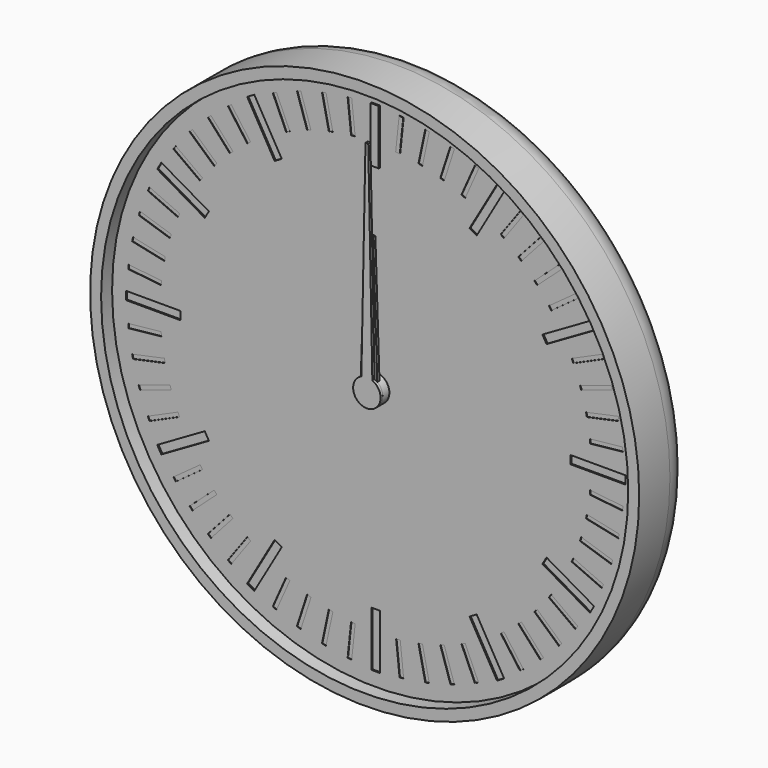
from build123d import *

# Parameters (mm, degrees)
F0_R      = 100
F1_DEPTH  = 24
F2_R      = 10
F3_T      = -4
F4_R      = 5
F4_R_2    = 3
F5_DEPTH  = 2
F6_DEPTH  = 19
F7_DEPTH  = 8
F9_DEPTH  = 4
F11_DEPTH = 4
F12_R     = 5
F12_R_2   = 3
F13_DEPTH = 2
F14_R     = 3
F15_DEPTH = 4
F17_DEPTH = 4
F18_R     = 3
F19_DEPTH = 2
F20_R     = 98
F20_R_2   = 5
F21_DEPTH = 1
F23_R     = 5
F23_R_2   = 3
F24_DEPTH = 2
F25_W     = 3
F25_H     = 20
F25_W_2   = 20
F25_H_2   = 3
F26_DEPTH = 0.5
F27_W     = 1.5
F27_H     = 12
F27_W_2   = 12
F27_H_2   = 1.5
F28_DEPTH = 0.2
F29_DEPTH = 1
F30_DEPTH = 0.4
F31_R     = 5
F31_R_2   = 3
F32_DEPTH = 5
F33_R     = 3
F34_DEPTH = 1
F36_DEPTH = 1


with BuildPart() as f1:
    # F0 (on Front) → F1 (new body)
    with BuildSketch(Plane.XZ):
        Circle(F0_R)
    extrude(amount=F1_DEPTH)

    # F2
    f2_edges = [f1.edges().sort_by_distance(p)[0] for p in [
        (-100, 0, 0),
    ]]
    fillet(f2_edges, radius=F2_R)

    # F3
    f3_openings = [f1.faces().sort_by_distance(p)[0] for p in [
        (0, -24, 0),
    ]]
    offset(amount=F3_T, openings=f3_openings)

    # F4 (on face) → F5 (join)
    with BuildSketch(Plane.XZ.offset(4)):
        Circle(F4_R)
        Circle(F4_R_2, mode=Mode.SUBTRACT)
        with Locations((40, 0)):
            Circle(F4_R)
        with Locations((40, 0)):
            Circle(F4_R_2, mode=Mode.SUBTRACT)
    extrude(amount=F5_DEPTH)


with BuildPart() as f6:
    # F6 (new): a face of the model
    f6_faces = [f1.part.faces().sort_by_distance(p)[0] for p in [
        (0, -4, 0),
    ]]
    extrude(f6_faces, amount=F6_DEPTH)

    # F8 (on face) → F9 (join)
    with BuildSketch(Plane.XZ.offset(6)):
        with BuildLine():
            ThreePointArc((9.2729637667, -1.3794085621), (9.3494561423, -0.6915886375), (9.375, 0))
            ThreePointArc((9.375, 0), (9.3494561423, 0.6915886375), (9.2729637667, 1.3794085621))
            ThreePointArc((9.2729637667, 1.3794085621), (8.9161548403, 2.8970343223), (8.3127812852, 4.3345463782))
            ThreePointArc((8.3127812852, 4.3345463782), (7.5845343223, 5.5104867402), (6.6911892658, 6.566476316))
            ThreePointArc((6.6911892658, 6.566476316), (5.5104867402, 7.5845343223), (4.1773988938, 8.3928519278))
            ThreePointArc((4.1773988938, 8.3928519278), (2.8970343223, 8.9161548403), (1.5536078905, 9.2453733036))
            ThreePointArc((1.5536078905, 9.2453733036), (0, 9.375), (-1.5536078905, 9.2453733036))
            ThreePointArc((-1.5536078905, 9.2453733036), (-2.8970343223, 8.9161548403), (-4.1773988938, 8.3928519278))
            ThreePointArc((-4.1773988938, 8.3928519278), (-5.5104867402, 7.5845343223), (-6.6911892658, 6.566476316))
            ThreePointArc((-6.6911892658, 6.566476316), (-7.5845343223, 5.5104867402), (-8.3127812852, 4.3345463782))
            ThreePointArc((-8.3127812852, 4.3345463782), (-8.9161548403, 2.8970343223), (-9.2729637667, 1.3794085621))
            ThreePointArc((-9.2729637667, 1.3794085621), (-9.375, 0), (-9.2729637667, -1.3794085621))
            ThreePointArc((-9.2729637667, -1.3794085621), (-8.9161548403, -2.8970343223), (-8.3127812852, -4.3345463782))
            ThreePointArc((-8.3127812852, -4.3345463782), (-7.5845343223, -5.5104867402), (-6.6911892658, -6.566476316))
            ThreePointArc((-6.6911892658, -6.566476316), (-5.5104867402, -7.5845343223), (-4.1773988938, -8.3928519278))
            ThreePointArc((-4.1773988938, -8.3928519278), (-2.8970343223, -8.9161548403), (-1.5536078905, -9.2453733036))
            ThreePointArc((-1.5536078905, -9.2453733036), (0, -9.375), (1.5536078905, -9.2453733036))
            ThreePointArc((1.5536078905, -9.2453733036), (2.8970343223, -8.9161548403), (4.1773988938, -8.3928519278))
            ThreePointArc((4.1773988938, -8.3928519278), (5.5104867402, -7.5845343223), (6.6911892658, -6.566476316))
            ThreePointArc((6.6911892658, -6.566476316), (7.5845343223, -5.5104867402), (8.3127812852, -4.3345463782))
            ThreePointArc((8.3127812852, -4.3345463782), (8.9161548403, -2.8970343223), (9.2729637667, -1.3794085621))
        make_face()
        with BuildLine():
            ThreePointArc((8.3127812852, 4.3345463782), (8.9161548403, 2.8970343223), (9.2729637667, 1.3794085621))
            Line((9.2729637667, 1.3794085621), (11.1823199426, 2.3946312492))
            Line((11.1823199426, 2.3946312492), (10.8182678729, 3.515068311))
            Line((10.8182678729, 3.515068311), (10.4542158031, 4.6355053728))
            Line((10.4542158031, 4.6355053728), (8.3127812852, 4.3345463782))
        make_face()
        with BuildLine():
            Line((11.1823199426, -2.3946312492), (9.2729637667, -1.3794085621))
            ThreePointArc((9.2729637667, -1.3794085621), (8.9161548403, -2.8970343223), (8.3127812852, -4.3345463782))
            Line((8.3127812852, -4.3345463782), (10.4542158031, -4.6355053728))
            Line((10.4542158031, -4.6355053728), (10.8182678729, -3.515068311))
            Line((10.8182678729, -3.515068311), (11.1823199426, -2.3946312492))
        make_face()
        with BuildLine():
            ThreePointArc((4.1773988938, 8.3928519278), (5.5104867402, 7.5845343223), (6.6911892658, 6.566476316))
            Line((6.6911892658, 6.566476316), (7.6391579371, 8.5101001246))
            Line((7.6391579371, 8.5101001246), (6.6860572448, 9.202568311))
            Line((6.6860572448, 9.202568311), (5.7329565525, 9.8950364974))
            Line((5.7329565525, 9.8950364974), (4.1773988938, 8.3928519278))
        make_face()
        with BuildLine():
            Line((7.6391579371, -8.5101001246), (6.6911892658, -6.566476316))
            ThreePointArc((6.6911892658, -6.566476316), (5.5104867402, -7.5845343223), (4.1773988938, -8.3928519278))
            Line((4.1773988938, -8.3928519278), (5.7329565525, -9.8950364974))
            Line((5.7329565525, -9.8950364974), (6.6860572448, -9.202568311))
            Line((6.6860572448, -9.202568311), (7.6391579371, -8.5101001246))
        make_face()
        with BuildLine():
            ThreePointArc((-1.5536078905, 9.2453733036), (0, 9.375), (1.5536078905, 9.2453733036))
            Line((1.5536078905, 9.2453733036), (1.1780972451, 11.375))
            Line((1.1780972451, 11.375), (0, 11.375))
            Line((0, 11.375), (-1.1780972451, 11.375))
            Line((-1.1780972451, 11.375), (-1.5536078905, 9.2453733036))
        make_face()
        with BuildLine():
            Line((1.1780972451, -11.375), (1.5536078905, -9.2453733036))
            ThreePointArc((1.5536078905, -9.2453733036), (0, -9.375), (-1.5536078905, -9.2453733036))
            Line((-1.5536078905, -9.2453733036), (-1.1780972451, -11.375))
            Line((-1.1780972451, -11.375), (0, -11.375))
            Line((0, -11.375), (1.1780972451, -11.375))
        make_face()
        with BuildLine():
            ThreePointArc((-6.6911892658, 6.566476316), (-5.5104867402, 7.5845343223), (-4.1773988938, 8.3928519278))
            Line((-4.1773988938, 8.3928519278), (-5.7329565525, 9.8950364974))
            Line((-5.7329565525, 9.8950364974), (-6.6860572448, 9.202568311))
            Line((-6.6860572448, 9.202568311), (-7.6391579371, 8.5101001246))
            Line((-7.6391579371, 8.5101001246), (-6.6911892658, 6.566476316))
        make_face()
        with BuildLine():
            Line((-5.7329565525, -9.8950364974), (-4.1773988938, -8.3928519278))
            ThreePointArc((-4.1773988938, -8.3928519278), (-5.5104867402, -7.5845343223), (-6.6911892658, -6.566476316))
            Line((-6.6911892658, -6.566476316), (-7.6391579371, -8.5101001246))
            Line((-7.6391579371, -8.5101001246), (-6.6860572448, -9.202568311))
            Line((-6.6860572448, -9.202568311), (-5.7329565525, -9.8950364974))
        make_face()
        with BuildLine():
            ThreePointArc((-9.2729637667, 1.3794085621), (-8.9161548403, 2.8970343223), (-8.3127812852, 4.3345463782))
            Line((-8.3127812852, 4.3345463782), (-10.4542158031, 4.6355053728))
            Line((-10.4542158031, 4.6355053728), (-10.8182678729, 3.515068311))
            Line((-10.8182678729, 3.515068311), (-11.1823199426, 2.3946312492))
            Line((-11.1823199426, 2.3946312492), (-9.2729637667, 1.3794085621))
        make_face()
        with BuildLine():
            Line((-10.4542158031, -4.6355053728), (-8.3127812852, -4.3345463782))
            ThreePointArc((-8.3127812852, -4.3345463782), (-8.9161548403, -2.8970343223), (-9.2729637667, -1.3794085621))
            Line((-9.2729637667, -1.3794085621), (-11.1823199426, -2.3946312492))
            Line((-11.1823199426, -2.3946312492), (-10.8182678729, -3.515068311))
            Line((-10.8182678729, -3.515068311), (-10.4542158031, -4.6355053728))
        make_face()
    extrude(amount=F9_DEPTH)

    # F35 (on face) → F36 (join)
    with BuildSketch(Plane.XZ.offset(23)):
        with BuildLine():
            ThreePointArc((-2, 4.582575695), (-2.7386127875, -4.1833001327), (5, 0))
            ThreePointArc((5, 0), (4.1833001327, 2.7386127875), (2, 4.582575695))
            ThreePointArc((2, 4.582575695), (0, 5), (-2, 4.582575695))
        make_face()
        with BuildLine():
            ThreePointArc((-2, 4.582575695), (0, 5), (2, 4.582575695))
            Line((2, 4.582575695), (0.5, 80))
            Line((0.5, 80), (0, 80))
            Line((0, 80), (-0.5, 80))
            Line((-0.5, 80), (-2, 4.582575695))
        make_face()
    extrude(amount=-F36_DEPTH)


with BuildPart() as f7:
    # F7 (new): a face of the model
    f7_faces = [f1.part.faces().sort_by_distance(p)[0] for p in [
        (40, -4, 0),
    ]]
    extrude(f7_faces, amount=F7_DEPTH)

    # F10 (on face) → F11 (join)
    with BuildSketch(Plane.XZ.offset(6)):
        with BuildLine():
            ThreePointArc((68.0829066802, -1.5381733945), (68.1144747006, -0.7693746225), (68.125, 0))
            ThreePointArc((68.125, 0), (68.1144747006, 0.7693746225), (68.0829066802, 1.5381733945))
            ThreePointArc((68.0829066802, 1.5381733945), (67.9709283072, 2.9398630294), (67.7890320221, 4.3342039956))
            ThreePointArc((67.7890320221, 4.3342039956), (67.5104012706, 5.8475163042), (67.1494235596, 7.3433252263))
            ThreePointArc((67.1494235596, 7.3433252263), (66.7484645208, 8.6911029668), (66.280643318, 10.0171558733))
            ThreePointArc((66.280643318, 10.0171558733), (65.6934659962, 11.4394680865), (65.0293803521, 12.8275385085))
            ThreePointArc((65.0293803521, 12.8275385085), (64.3569644814, 14.0625), (63.6236643925, 15.2623099717))
            ThreePointArc((63.6236643925, 15.2623099717), (62.7536029668, 16.5314602207), (61.815433119, 17.7511268046))
            ThreePointArc((61.815433119, 17.7511268046), (60.9009482166, 18.8192983038), (59.934217974, 19.8404278876))
            ThreePointArc((59.934217974, 19.8404278876), (58.8192983038, 20.9009482166), (57.6480467764, 21.8989056799))
            ThreePointArc((57.6480467764, 21.8989056799), (56.5314602207, 22.7536029668), (55.3735505752, 23.5514238999))
            ThreePointArc((55.3735505752, 23.5514238999), (54.0625, 24.3569644814), (52.709356105, 25.0895972944))
            ThreePointArc((52.709356105, 25.0895972944), (51.4394680865, 25.6934659962), (50.1409852457, 26.2331096755))
            ThreePointArc((50.1409852457, 26.2331096755), (48.6911029668, 26.7484645208), (47.2152055856, 27.1837531139))
            ThreePointArc((47.2152055856, 27.1837531139), (45.8475163042, 27.5104012706), (44.4652101991, 27.7682826779))
            ThreePointArc((44.4652101991, 27.7682826779), (42.9398630294, 27.9709283072), (41.4057159597, 28.0898484802))
            ThreePointArc((41.4057159597, 28.0898484802), (40, 28.125), (38.5942840403, 28.0898484802))
            ThreePointArc((38.5942840403, 28.0898484802), (37.0601369706, 27.9709283072), (35.5347898009, 27.7682826779))
            ThreePointArc((35.5347898009, 27.7682826779), (34.1524836958, 27.5104012706), (32.7847944144, 27.1837531139))
            ThreePointArc((32.7847944144, 27.1837531139), (31.3088970332, 26.7484645208), (29.8590147543, 26.2331096755))
            ThreePointArc((29.8590147543, 26.2331096755), (28.5605319135, 25.6934659962), (27.290643895, 25.0895972944))
            ThreePointArc((27.290643895, 25.0895972944), (25.9375, 24.3569644814), (24.6264494248, 23.5514238999))
            ThreePointArc((24.6264494248, 23.5514238999), (23.4685397793, 22.7536029668), (22.3519532236, 21.8989056799))
            ThreePointArc((22.3519532236, 21.8989056799), (21.1807016962, 20.9009482166), (20.065782026, 19.8404278876))
            ThreePointArc((20.065782026, 19.8404278876), (19.0990517834, 18.8192983038), (18.184566881, 17.7511268046))
            ThreePointArc((18.184566881, 17.7511268046), (17.2463970332, 16.5314602207), (16.3763356075, 15.2623099717))
            ThreePointArc((16.3763356075, 15.2623099717), (15.6430355186, 14.0625), (14.9706196479, 12.8275385085))
            ThreePointArc((14.9706196479, 12.8275385085), (14.3065340038, 11.4394680865), (13.719356682, 10.0171558733))
            ThreePointArc((13.719356682, 10.0171558733), (13.2515354792, 8.6911029668), (12.8505764404, 7.3433252263))
            ThreePointArc((12.8505764404, 7.3433252263), (12.4895987294, 5.8475163042), (12.2109679779, 4.3342039956))
            ThreePointArc((12.2109679779, 4.3342039956), (12.0290716928, 2.9398630294), (11.9170933198, 1.5381733945))
            ThreePointArc((11.9170933198, 1.5381733945), (11.875, 0), (11.9170933198, -1.5381733945))
            ThreePointArc((11.9170933198, -1.5381733945), (12.0290716928, -2.9398630294), (12.2109679779, -4.3342039956))
            ThreePointArc((12.2109679779, -4.3342039956), (12.4895987294, -5.8475163042), (12.8505764404, -7.3433252263))
            ThreePointArc((12.8505764404, -7.3433252263), (13.2515354792, -8.6911029668), (13.719356682, -10.0171558733))
            ThreePointArc((13.719356682, -10.0171558733), (14.3065340038, -11.4394680865), (14.9706196479, -12.8275385085))
            ThreePointArc((14.9706196479, -12.8275385085), (15.6430355186, -14.0625), (16.3763356075, -15.2623099717))
            ThreePointArc((16.3763356075, -15.2623099717), (17.2463970332, -16.5314602207), (18.184566881, -17.7511268046))
            ThreePointArc((18.184566881, -17.7511268046), (19.0990517834, -18.8192983038), (20.065782026, -19.8404278876))
            ThreePointArc((20.065782026, -19.8404278876), (21.1807016962, -20.9009482166), (22.3519532236, -21.8989056799))
            ThreePointArc((22.3519532236, -21.8989056799), (23.4685397793, -22.7536029668), (24.6264494248, -23.5514238999))
            ThreePointArc((24.6264494248, -23.5514238999), (25.9375, -24.3569644814), (27.290643895, -25.0895972944))
            ThreePointArc((27.290643895, -25.0895972944), (28.5605319135, -25.6934659962), (29.8590147543, -26.2331096755))
            ThreePointArc((29.8590147543, -26.2331096755), (31.3088970332, -26.7484645208), (32.7847944144, -27.1837531139))
            ThreePointArc((32.7847944144, -27.1837531139), (34.1524836958, -27.5104012706), (35.5347898009, -27.7682826779))
            ThreePointArc((35.5347898009, -27.7682826779), (37.0601369706, -27.9709283072), (38.5942840403, -28.0898484802))
            ThreePointArc((38.5942840403, -28.0898484802), (40, -28.125), (41.4057159597, -28.0898484802))
            ThreePointArc((41.4057159597, -28.0898484802), (42.9398630294, -27.9709283072), (44.4652101991, -27.7682826779))
            ThreePointArc((44.4652101991, -27.7682826779), (45.8475163042, -27.5104012706), (47.2152055856, -27.1837531139))
            ThreePointArc((47.2152055856, -27.1837531139), (48.6911029668, -26.7484645208), (50.1409852457, -26.2331096755))
            ThreePointArc((50.1409852457, -26.2331096755), (51.4394680865, -25.6934659962), (52.709356105, -25.0895972944))
            ThreePointArc((52.709356105, -25.0895972944), (54.0625, -24.3569644814), (55.3735505752, -23.5514238999))
            ThreePointArc((55.3735505752, -23.5514238999), (56.5314602207, -22.7536029668), (57.6480467764, -21.8989056799))
            ThreePointArc((57.6480467764, -21.8989056799), (58.8192983038, -20.9009482166), (59.934217974, -19.8404278876))
            ThreePointArc((59.934217974, -19.8404278876), (60.9009482166, -18.8192983038), (61.815433119, -17.7511268046))
            ThreePointArc((61.815433119, -17.7511268046), (62.7536029668, -16.5314602207), (63.6236643925, -15.2623099717))
            ThreePointArc((63.6236643925, -15.2623099717), (64.3569644814, -14.0625), (65.0293803521, -12.8275385085))
            ThreePointArc((65.0293803521, -12.8275385085), (65.6934659962, -11.4394680865), (66.280643318, -10.0171558733))
            ThreePointArc((66.280643318, -10.0171558733), (66.7484645208, -8.6911029668), (67.1494235596, -7.3433252263))
            ThreePointArc((67.1494235596, -7.3433252263), (67.5104012706, -5.8475163042), (67.7890320221, -4.3342039956))
            ThreePointArc((67.7890320221, -4.3342039956), (67.9709283072, -2.9398630294), (68.0829066802, -1.5381733945))
        make_face()
        with BuildLine():
            ThreePointArc((68.0829066802, 1.5381733945), (68.1144747006, 0.7693746225), (68.125, 0))
            ThreePointArc((68.125, 0), (68.1144747006, -0.7693746225), (68.0829066802, -1.5381733945))
            Line((68.0829066802, -1.5381733945), (70.125, -1.1780972451))
            Line((70.125, -1.1780972451), (70.125, 0))
            Line((70.125, 0), (70.125, 1.1780972451))
            Line((70.125, 1.1780972451), (68.0829066802, 1.5381733945))
        make_face()
        with BuildLine():
            ThreePointArc((67.1494235596, 7.3433252263), (67.5104012706, 5.8475163042), (67.7890320221, 4.3342039956))
            Line((67.7890320221, 4.3342039956), (69.7116366623, 5.1109866922))
            Line((69.7116366623, 5.1109866922), (69.4666964721, 6.2633396859))
            Line((69.4666964721, 6.2633396859), (69.2217562819, 7.4156926796))
            Line((69.2217562819, 7.4156926796), (67.1494235596, 7.3433252263))
        make_face()
        with BuildLine():
            Line((69.7116366623, -5.1109866922), (67.7890320221, -4.3342039956))
            ThreePointArc((67.7890320221, -4.3342039956), (67.5104012706, -5.8475163042), (67.1494235596, -7.3433252263))
            Line((67.1494235596, -7.3433252263), (69.2217562819, -7.4156926796))
            Line((69.2217562819, -7.4156926796), (69.4666964721, -6.2633396859))
            Line((69.4666964721, -6.2633396859), (69.7116366623, -5.1109866922))
        make_face()
        with BuildLine():
            ThreePointArc((65.0293803521, 12.8275385085), (65.6934659962, 11.4394680865), (66.280643318, 10.0171558733))
            Line((66.280643318, 10.0171558733), (67.9997322302, 11.1766959857))
            Line((67.9997322302, 11.1766959857), (67.5205569115, 12.2529413727))
            Line((67.5205569115, 12.2529413727), (67.0413815928, 13.3291867596))
            Line((67.0413815928, 13.3291867596), (65.0293803521, 12.8275385085))
        make_face()
        with BuildLine():
            Line((67.9997322302, -11.1766959857), (66.280643318, -10.0171558733))
            ThreePointArc((66.280643318, -10.0171558733), (65.6934659962, -11.4394680865), (65.0293803521, -12.8275385085))
            Line((65.0293803521, -12.8275385085), (67.0413815928, -13.3291867596))
            Line((67.0413815928, -13.3291867596), (67.5205569115, -12.2529413727))
            Line((67.5205569115, -12.2529413727), (67.9997322302, -11.1766959857))
        make_face()
        with BuildLine():
            ThreePointArc((61.815433119, 17.7511268046), (62.7536029668, 16.5314602207), (63.6236643925, 15.2623099717))
            Line((63.6236643925, 15.2623099717), (65.064105142, 16.753930033))
            Line((65.064105142, 16.753930033), (64.3716369555, 17.7070307253))
            Line((64.3716369555, 17.7070307253), (63.6791687691, 18.6601314176))
            Line((63.6791687691, 18.6601314176), (61.815433119, 17.7511268046))
        make_face()
        with BuildLine():
            Line((65.064105142, -16.753930033), (63.6236643925, -15.2623099717))
            ThreePointArc((63.6236643925, -15.2623099717), (62.7536029668, -16.5314602207), (61.815433119, -17.7511268046))
            Line((61.815433119, -17.7511268046), (63.6791687691, -18.6601314176))
            Line((63.6791687691, -18.6601314176), (64.3716369555, -17.7070307253))
            Line((64.3716369555, -17.7070307253), (65.064105142, -16.753930033))
        make_face()
        with BuildLine():
            ThreePointArc((57.6480467764, 21.8989056799), (58.8192983038, 20.9009482166), (59.934217974, 19.8404278876))
            Line((59.934217974, 19.8404278876), (61.0330563882, 21.5989369435))
            Line((61.0330563882, 21.5989369435), (60.1575595166, 22.3872378675))
            Line((60.1575595166, 22.3872378675), (59.282062645, 23.1755387915))
            Line((59.282062645, 23.1755387915), (57.6480467764, 21.8989056799))
        make_face()
        with BuildLine():
            Line((61.0330563882, -21.5989369435), (59.934217974, -19.8404278876))
            ThreePointArc((59.934217974, -19.8404278876), (58.8192983038, -20.9009482166), (57.6480467764, -21.8989056799))
            Line((57.6480467764, -21.8989056799), (59.282062645, -23.1755387915))
            Line((59.282062645, -23.1755387915), (60.1575595166, -22.3872378675))
            Line((60.1575595166, -22.3872378675), (61.0330563882, -21.5989369435))
        make_face()
        with BuildLine():
            ThreePointArc((52.709356105, 25.0895972944), (54.0625, 24.3569644814), (55.3735505752, 23.5514238999))
            Line((55.3735505752, 23.5514238999), (56.0827621424, 25.4999666665))
            Line((56.0827621424, 25.4999666665), (55.0625, 26.089015289))
            Line((55.0625, 26.089015289), (54.0422378576, 26.6780639116))
            Line((54.0422378576, 26.6780639116), (52.709356105, 25.0895972944))
        make_face()
        with BuildLine():
            Line((56.0827621424, -25.4999666665), (55.3735505752, -23.5514238999))
            ThreePointArc((55.3735505752, -23.5514238999), (54.0625, -24.3569644814), (52.709356105, -25.0895972944))
            Line((52.709356105, -25.0895972944), (54.0422378576, -26.6780639116))
            Line((54.0422378576, -26.6780639116), (55.0625, -26.089015289))
            Line((55.0625, -26.089015289), (56.0827621424, -25.4999666665))
        make_face()
        with BuildLine():
            ThreePointArc((47.2152055856, 27.1837531139), (48.6911029668, 26.7484645208), (50.1409852457, 26.2331096755))
            Line((50.1409852457, 26.2331096755), (50.4295740173, 28.2865254836))
            Line((50.4295740173, 28.2865254836), (49.3091369555, 28.6505775534))
            Line((49.3091369555, 28.6505775534), (48.1886998938, 29.0146296232))
            Line((48.1886998938, 29.0146296232), (47.2152055856, 27.1837531139))
        make_face()
        with BuildLine():
            Line((50.4295740173, -28.2865254836), (50.1409852457, -26.2331096755))
            ThreePointArc((50.1409852457, -26.2331096755), (48.6911029668, -26.7484645208), (47.2152055856, -27.1837531139))
            Line((47.2152055856, -27.1837531139), (48.1886998938, -29.0146296232))
            Line((48.1886998938, -29.0146296232), (49.3091369555, -28.6505775534))
            Line((49.3091369555, -28.6505775534), (50.4295740173, -28.2865254836))
        make_face()
        with BuildLine():
            ThreePointArc((41.4057159597, 28.0898484802), (42.9398630294, 27.9709283072), (44.4652101991, 27.7682826779))
            Line((44.4652101991, 27.7682826779), (44.3205634611, 29.8368274034))
            Line((44.3205634611, 29.8368274034), (43.1489199559, 29.959972098))
            Line((43.1489199559, 29.959972098), (41.9772764508, 30.0831167926))
            Line((41.9772764508, 30.0831167926), (41.4057159597, 28.0898484802))
        make_face()
        with BuildLine():
            Line((44.3205634611, -29.8368274034), (44.4652101991, -27.7682826779))
            ThreePointArc((44.4652101991, -27.7682826779), (42.9398630294, -27.9709283072), (41.4057159597, -28.0898484802))
            Line((41.4057159597, -28.0898484802), (41.9772764508, -30.0831167926))
            Line((41.9772764508, -30.0831167926), (43.1489199559, -29.959972098))
            Line((43.1489199559, -29.959972098), (44.3205634611, -29.8368274034))
        make_face()
        with BuildLine():
            ThreePointArc((35.5347898009, 27.7682826779), (37.0601369706, 27.9709283072), (38.5942840403, 28.0898484802))
            Line((38.5942840403, 28.0898484802), (38.0227235492, 30.0831167926))
            Line((38.0227235492, 30.0831167926), (36.8510800441, 29.959972098))
            Line((36.8510800441, 29.959972098), (35.6794365389, 29.8368274034))
            Line((35.6794365389, 29.8368274034), (35.5347898009, 27.7682826779))
        make_face()
        with BuildLine():
            Line((38.0227235492, -30.0831167926), (38.5942840403, -28.0898484802))
            ThreePointArc((38.5942840403, -28.0898484802), (37.0601369706, -27.9709283072), (35.5347898009, -27.7682826779))
            Line((35.5347898009, -27.7682826779), (35.6794365389, -29.8368274034))
            Line((35.6794365389, -29.8368274034), (36.8510800441, -29.959972098))
            Line((36.8510800441, -29.959972098), (38.0227235492, -30.0831167926))
        make_face()
        with BuildLine():
            ThreePointArc((29.8590147543, 26.2331096755), (31.3088970332, 26.7484645208), (32.7847944144, 27.1837531139))
            Line((32.7847944144, 27.1837531139), (31.8113001062, 29.0146296232))
            Line((31.8113001062, 29.0146296232), (30.6908630445, 28.6505775534))
            Line((30.6908630445, 28.6505775534), (29.5704259827, 28.2865254836))
            Line((29.5704259827, 28.2865254836), (29.8590147543, 26.2331096755))
        make_face()
        with BuildLine():
            Line((31.8113001062, -29.0146296232), (32.7847944144, -27.1837531139))
            ThreePointArc((32.7847944144, -27.1837531139), (31.3088970332, -26.7484645208), (29.8590147543, -26.2331096755))
            Line((29.8590147543, -26.2331096755), (29.5704259827, -28.2865254836))
            Line((29.5704259827, -28.2865254836), (30.6908630445, -28.6505775534))
            Line((30.6908630445, -28.6505775534), (31.8113001062, -29.0146296232))
        make_face()
        with BuildLine():
            ThreePointArc((24.6264494248, 23.5514238999), (25.9375, 24.3569644814), (27.290643895, 25.0895972944))
            Line((27.290643895, 25.0895972944), (25.9577621424, 26.6780639116))
            Line((25.9577621424, 26.6780639116), (24.9375, 26.089015289))
            Line((24.9375, 26.089015289), (23.9172378576, 25.4999666665))
            Line((23.9172378576, 25.4999666665), (24.6264494248, 23.5514238999))
        make_face()
        with BuildLine():
            Line((25.9577621424, -26.6780639116), (27.290643895, -25.0895972944))
            ThreePointArc((27.290643895, -25.0895972944), (25.9375, -24.3569644814), (24.6264494248, -23.5514238999))
            Line((24.6264494248, -23.5514238999), (23.9172378576, -25.4999666665))
            Line((23.9172378576, -25.4999666665), (24.9375, -26.089015289))
            Line((24.9375, -26.089015289), (25.9577621424, -26.6780639116))
        make_face()
        with BuildLine():
            ThreePointArc((20.065782026, 19.8404278876), (21.1807016962, 20.9009482166), (22.3519532236, 21.8989056799))
            Line((22.3519532236, 21.8989056799), (20.717937355, 23.1755387915))
            Line((20.717937355, 23.1755387915), (19.8424404834, 22.3872378675))
            Line((19.8424404834, 22.3872378675), (18.9669436118, 21.5989369435))
            Line((18.9669436118, 21.5989369435), (20.065782026, 19.8404278876))
        make_face()
        with BuildLine():
            Line((20.717937355, -23.1755387915), (22.3519532236, -21.8989056799))
            ThreePointArc((22.3519532236, -21.8989056799), (21.1807016962, -20.9009482166), (20.065782026, -19.8404278876))
            Line((20.065782026, -19.8404278876), (18.9669436118, -21.5989369435))
            Line((18.9669436118, -21.5989369435), (19.8424404834, -22.3872378675))
            Line((19.8424404834, -22.3872378675), (20.717937355, -23.1755387915))
        make_face()
        with BuildLine():
            ThreePointArc((16.3763356075, 15.2623099717), (17.2463970332, 16.5314602207), (18.184566881, 17.7511268046))
            Line((18.184566881, 17.7511268046), (16.3208312309, 18.6601314176))
            Line((16.3208312309, 18.6601314176), (15.6283630445, 17.7070307253))
            Line((15.6283630445, 17.7070307253), (14.935894858, 16.753930033))
            Line((14.935894858, 16.753930033), (16.3763356075, 15.2623099717))
        make_face()
        with BuildLine():
            Line((16.3208312309, -18.6601314176), (18.184566881, -17.7511268046))
            ThreePointArc((18.184566881, -17.7511268046), (17.2463970332, -16.5314602207), (16.3763356075, -15.2623099717))
            Line((16.3763356075, -15.2623099717), (14.935894858, -16.753930033))
            Line((14.935894858, -16.753930033), (15.6283630445, -17.7070307253))
            Line((15.6283630445, -17.7070307253), (16.3208312309, -18.6601314176))
        make_face()
        with BuildLine():
            ThreePointArc((13.719356682, 10.0171558733), (14.3065340038, 11.4394680865), (14.9706196479, 12.8275385085))
            Line((14.9706196479, 12.8275385085), (12.9586184072, 13.3291867596))
            Line((12.9586184072, 13.3291867596), (12.4794430885, 12.2529413727))
            Line((12.4794430885, 12.2529413727), (12.0002677698, 11.1766959857))
            Line((12.0002677698, 11.1766959857), (13.719356682, 10.0171558733))
        make_face()
        with BuildLine():
            Line((12.9586184072, -13.3291867596), (14.9706196479, -12.8275385085))
            ThreePointArc((14.9706196479, -12.8275385085), (14.3065340038, -11.4394680865), (13.719356682, -10.0171558733))
            Line((13.719356682, -10.0171558733), (12.0002677698, -11.1766959857))
            Line((12.0002677698, -11.1766959857), (12.4794430885, -12.2529413727))
            Line((12.4794430885, -12.2529413727), (12.9586184072, -13.3291867596))
        make_face()
        with BuildLine():
            ThreePointArc((12.2109679779, 4.3342039956), (12.4895987294, 5.8475163042), (12.8505764404, 7.3433252263))
            Line((12.8505764404, 7.3433252263), (10.7782437181, 7.4156926796))
            Line((10.7782437181, 7.4156926796), (10.5333035279, 6.2633396859))
            Line((10.5333035279, 6.2633396859), (10.2883633377, 5.1109866922))
            Line((10.2883633377, 5.1109866922), (12.2109679779, 4.3342039956))
        make_face()
        with BuildLine():
            Line((10.7782437181, -7.4156926796), (12.8505764404, -7.3433252263))
            ThreePointArc((12.8505764404, -7.3433252263), (12.4895987294, -5.8475163042), (12.2109679779, -4.3342039956))
            Line((12.2109679779, -4.3342039956), (10.2883633377, -5.1109866922))
            Line((10.2883633377, -5.1109866922), (10.5333035279, -6.2633396859))
            Line((10.5333035279, -6.2633396859), (10.7782437181, -7.4156926796))
        make_face()
        with BuildLine():
            ThreePointArc((11.9170933198, -1.5381733945), (11.875, 0), (11.9170933198, 1.5381733945))
            Line((11.9170933198, 1.5381733945), (9.875, 1.1780972451))
            Line((9.875, 1.1780972451), (9.875, 0))
            Line((9.875, 0), (9.875, -1.1780972451))
            Line((9.875, -1.1780972451), (11.9170933198, -1.5381733945))
        make_face()
    extrude(amount=F11_DEPTH)

    # F16 (on face) → F17 (join)
    with BuildSketch(Plane.XZ.offset(12)):
        with BuildLine():
            ThreePointArc((47.4288750323, -1.0304444454), (47.4821976298, -0.5164480894), (47.5, 0))
            ThreePointArc((47.5, 0), (47.4821976298, 0.5164480894), (47.4288750323, 1.0304444454))
            ThreePointArc((47.4288750323, 1.0304444454), (47.1329238722, 2.3176274578), (46.6157661985, 3.532936117))
            ThreePointArc((46.6157661985, 3.532936117), (46.0676274578, 4.4083893922), (45.4044061018, 5.2002302532))
            ThreePointArc((45.4044061018, 5.2002302532), (44.4083893922, 6.0676274578), (43.2756595386, 6.7468551628))
            ThreePointArc((43.2756595386, 6.7468551628), (42.3176274578, 7.1329238722), (41.3156377295, 7.3837048536))
            ThreePointArc((41.3156377295, 7.3837048536), (40, 7.5), (38.6843622705, 7.3837048536))
            ThreePointArc((38.6843622705, 7.3837048536), (37.6823725422, 7.1329238722), (36.7243404614, 6.7468551628))
            ThreePointArc((36.7243404614, 6.7468551628), (35.5916106078, 6.0676274578), (34.5955938982, 5.2002302532))
            ThreePointArc((34.5955938982, 5.2002302532), (33.9323725422, 4.4083893922), (33.3842338015, 3.532936117))
            ThreePointArc((33.3842338015, 3.532936117), (32.8670761278, 2.3176274578), (32.5711249677, 1.0304444454))
            ThreePointArc((32.5711249677, 1.0304444454), (32.5, 0), (32.5711249677, -1.0304444454))
            ThreePointArc((32.5711249677, -1.0304444454), (32.8670761278, -2.3176274578), (33.3842338015, -3.532936117))
            ThreePointArc((33.3842338015, -3.532936117), (33.9323725422, -4.4083893922), (34.5955938982, -5.2002302532))
            ThreePointArc((34.5955938982, -5.2002302532), (35.5916106078, -6.0676274578), (36.7243404614, -6.7468551628))
            ThreePointArc((36.7243404614, -6.7468551628), (37.6823725422, -7.1329238722), (38.6843622705, -7.3837048536))
            ThreePointArc((38.6843622705, -7.3837048536), (40, -7.5), (41.3156377295, -7.3837048536))
            ThreePointArc((41.3156377295, -7.3837048536), (42.3176274578, -7.1329238722), (43.2756595386, -6.7468551628))
            ThreePointArc((43.2756595386, -6.7468551628), (44.4083893922, -6.0676274578), (45.4044061018, -5.2002302532))
            ThreePointArc((45.4044061018, -5.2002302532), (46.0676274578, -4.4083893922), (46.6157661985, -3.532936117))
            ThreePointArc((46.6157661985, -3.532936117), (47.1329238722, -2.3176274578), (47.4288750323, -1.0304444454))
        make_face()
        with BuildLine():
            ThreePointArc((46.6157661985, 3.532936117), (47.1329238722, 2.3176274578), (47.4288750323, 1.0304444454))
            Line((47.4288750323, 1.0304444454), (49.3262785606, 2.0393117971))
            Line((49.3262785606, 2.0393117971), (48.743795249, 3.832011096))
            Line((48.743795249, 3.832011096), (46.6157661985, 3.532936117))
        make_face()
        with BuildLine():
            Line((49.3262785606, -2.0393117971), (47.4288750323, -1.0304444454))
            ThreePointArc((47.4288750323, -1.0304444454), (47.1329238722, -2.3176274578), (46.6157661985, -3.532936117))
            Line((46.6157661985, -3.532936117), (48.743795249, -3.832011096))
            Line((48.743795249, -3.832011096), (49.3262785606, -2.0393117971))
        make_face()
        with BuildLine():
            ThreePointArc((43.2756595386, 6.7468551628), (44.4083893922, 6.0676274578), (45.4044061018, 5.2002302532))
            Line((45.4044061018, 5.2002302532), (46.3464404506, 7.1316868974))
            Line((46.3464404506, 7.1316868974), (44.8214793429, 8.2396359957))
            Line((44.8214793429, 8.2396359957), (43.2756595386, 6.7468551628))
        make_face()
        with BuildLine():
            Line((46.3464404506, -7.1316868974), (45.4044061018, -5.2002302532))
            ThreePointArc((45.4044061018, -5.2002302532), (44.4083893922, -6.0676274578), (43.2756595386, -6.7468551628))
            Line((43.2756595386, -6.7468551628), (44.8214793429, -8.2396359957))
            Line((44.8214793429, -8.2396359957), (46.3464404506, -7.1316868974))
        make_face()
        with BuildLine():
            ThreePointArc((38.6843622705, 7.3837048536), (40, 7.5), (41.3156377295, 7.3837048536))
            Line((41.3156377295, 7.3837048536), (40.9424777961, 9.5))
            Line((40.9424777961, 9.5), (39.0575222039, 9.5))
            Line((39.0575222039, 9.5), (38.6843622705, 7.3837048536))
        make_face()
        with BuildLine():
            Line((40.9424777961, -9.5), (41.3156377295, -7.3837048536))
            ThreePointArc((41.3156377295, -7.3837048536), (40, -7.5), (38.6843622705, -7.3837048536))
            Line((38.6843622705, -7.3837048536), (39.0575222039, -9.5))
            Line((39.0575222039, -9.5), (40.9424777961, -9.5))
        make_face()
        with BuildLine():
            ThreePointArc((34.5955938982, 5.2002302532), (35.5916106078, 6.0676274578), (36.7243404614, 6.7468551628))
            Line((36.7243404614, 6.7468551628), (35.1785206571, 8.2396359957))
            Line((35.1785206571, 8.2396359957), (33.6535595494, 7.1316868974))
            Line((33.6535595494, 7.1316868974), (34.5955938982, 5.2002302532))
        make_face()
        with BuildLine():
            Line((35.1785206571, -8.2396359957), (36.7243404614, -6.7468551628))
            ThreePointArc((36.7243404614, -6.7468551628), (35.5916106078, -6.0676274578), (34.5955938982, -5.2002302532))
            Line((34.5955938982, -5.2002302532), (33.6535595494, -7.1316868974))
            Line((33.6535595494, -7.1316868974), (35.1785206571, -8.2396359957))
        make_face()
        with BuildLine():
            ThreePointArc((32.5711249677, 1.0304444454), (32.8670761278, 2.3176274578), (33.3842338015, 3.532936117))
            Line((33.3842338015, 3.532936117), (31.256204751, 3.832011096))
            Line((31.256204751, 3.832011096), (30.6737214394, 2.0393117971))
            Line((30.6737214394, 2.0393117971), (32.5711249677, 1.0304444454))
        make_face()
        with BuildLine():
            Line((31.256204751, -3.832011096), (33.3842338015, -3.532936117))
            ThreePointArc((33.3842338015, -3.532936117), (32.8670761278, -2.3176274578), (32.5711249677, -1.0304444454))
            Line((32.5711249677, -1.0304444454), (30.6737214394, -2.0393117971))
            Line((30.6737214394, -2.0393117971), (31.256204751, -3.832011096))
        make_face()
    extrude(amount=F17_DEPTH)

    # F18 (on face) → F19 (join)
    with BuildSketch(Plane.XZ.offset(16)):
        with Locations((40, 0)):
            Circle(F18_R)
    extrude(amount=F19_DEPTH)


with BuildPart() as f13:
    # F12 (on face) → F13 (new body)
    with BuildSketch(Plane.XZ.offset(10)):
        Circle(F12_R)
        Circle(F12_R_2, mode=Mode.SUBTRACT)
    extrude(amount=F13_DEPTH)

    # F14 (on face) → F15 (join)
    with BuildSketch(Plane.XZ.offset(12)):
        with BuildLine():
            ThreePointArc((29.9718156995, -1.3001014101), (29.9929530972, -0.6502034357), (30, 0))
            ThreePointArc((30, 0), (29.9929530972, 0.6502034357), (29.9718156995, 1.3001014101))
            ThreePointArc((29.9718156995, 1.3001014101), (29.907520012, 2.3537728718), (29.8061935814, 3.4045299509))
            ThreePointArc((29.8061935814, 3.4045299509), (29.6306502179, 4.6930339512), (29.3994322443, 5.9727199596))
            ThreePointArc((29.3994322443, 5.9727199596), (29.1710976119, 7.0033609157), (28.9066440563, 8.0253304855))
            ThreePointArc((28.9066440563, 8.0253304855), (28.5316954889, 9.2705098312), (28.1031371961, 10.4982703213))
            ThreePointArc((28.1031371961, 10.4982703213), (27.7163859753, 11.480502971), (27.2953170189, 12.448520749))
            ThreePointArc((27.2953170189, 12.448520749), (26.7301957257, 13.6197149922), (26.1148496411, 14.765318426))
            ThreePointArc((26.1148496411, 14.765318426), (25.5792049306, 15.6749569415), (25.0118886885, 16.5651871174))
            ThreePointArc((25.0118886885, 16.5651871174), (24.2705098312, 17.6335575688), (23.4835278178, 18.6687953878))
            ThreePointArc((23.4835278178, 18.6687953878), (22.812178968, 19.4834414499), (22.1125846489, 20.2739636023))
            ThreePointArc((22.1125846489, 20.2739636023), (21.2132034356, 21.2132034356), (20.2739636023, 22.1125846489))
            ThreePointArc((20.2739636023, 22.1125846489), (19.4834414499, 22.812178968), (18.6687953878, 23.4835278178))
            ThreePointArc((18.6687953878, 23.4835278178), (17.6335575688, 24.2705098312), (16.5651871174, 25.0118886885))
            ThreePointArc((16.5651871174, 25.0118886885), (15.6749569415, 25.5792049306), (14.765318426, 26.1148496411))
            ThreePointArc((14.765318426, 26.1148496411), (13.6197149922, 26.7301957257), (12.448520749, 27.2953170189))
            ThreePointArc((12.448520749, 27.2953170189), (11.480502971, 27.7163859753), (10.4982703213, 28.1031371961))
            ThreePointArc((10.4982703213, 28.1031371961), (9.2705098312, 28.5316954889), (8.0253304855, 28.9066440563))
            ThreePointArc((8.0253304855, 28.9066440563), (7.0033609157, 29.1710976119), (5.9727199596, 29.3994322443))
            ThreePointArc((5.9727199596, 29.3994322443), (4.6930339512, 29.6306502179), (3.4045299509, 29.8061935814))
            ThreePointArc((3.4045299509, 29.8061935814), (2.3537728718, 29.907520012), (1.3001014101, 29.9718156995))
            ThreePointArc((1.3001014101, 29.9718156995), (0, 30), (-1.3001014101, 29.9718156995))
            ThreePointArc((-1.3001014101, 29.9718156995), (-2.3537728718, 29.907520012), (-3.4045299509, 29.8061935814))
            ThreePointArc((-3.4045299509, 29.8061935814), (-4.6930339512, 29.6306502179), (-5.9727199596, 29.3994322443))
            ThreePointArc((-5.9727199596, 29.3994322443), (-7.0033609157, 29.1710976119), (-8.0253304855, 28.9066440563))
            ThreePointArc((-8.0253304855, 28.9066440563), (-9.2705098312, 28.5316954889), (-10.4982703213, 28.1031371961))
            ThreePointArc((-10.4982703213, 28.1031371961), (-11.480502971, 27.7163859753), (-12.448520749, 27.2953170189))
            ThreePointArc((-12.448520749, 27.2953170189), (-13.6197149922, 26.7301957257), (-14.765318426, 26.1148496411))
            ThreePointArc((-14.765318426, 26.1148496411), (-15.6749569415, 25.5792049306), (-16.5651871174, 25.0118886885))
            ThreePointArc((-16.5651871174, 25.0118886885), (-17.6335575688, 24.2705098312), (-18.6687953878, 23.4835278178))
            ThreePointArc((-18.6687953878, 23.4835278178), (-19.4834414499, 22.812178968), (-20.2739636023, 22.1125846489))
            ThreePointArc((-20.2739636023, 22.1125846489), (-21.2132034356, 21.2132034356), (-22.1125846489, 20.2739636023))
            ThreePointArc((-22.1125846489, 20.2739636023), (-22.812178968, 19.4834414499), (-23.4835278178, 18.6687953878))
            ThreePointArc((-23.4835278178, 18.6687953878), (-24.2705098312, 17.6335575688), (-25.0118886885, 16.5651871174))
            ThreePointArc((-25.0118886885, 16.5651871174), (-25.5792049306, 15.6749569415), (-26.1148496411, 14.765318426))
            ThreePointArc((-26.1148496411, 14.765318426), (-26.7301957257, 13.6197149922), (-27.2953170189, 12.448520749))
            ThreePointArc((-27.2953170189, 12.448520749), (-27.7163859753, 11.480502971), (-28.1031371961, 10.4982703213))
            ThreePointArc((-28.1031371961, 10.4982703213), (-28.5316954889, 9.2705098312), (-28.9066440563, 8.0253304855))
            ThreePointArc((-28.9066440563, 8.0253304855), (-29.1710976119, 7.0033609157), (-29.3994322443, 5.9727199596))
            ThreePointArc((-29.3994322443, 5.9727199596), (-29.6306502179, 4.6930339512), (-29.8061935814, 3.4045299509))
            ThreePointArc((-29.8061935814, 3.4045299509), (-29.907520012, 2.3537728718), (-29.9718156995, 1.3001014101))
            ThreePointArc((-29.9718156995, 1.3001014101), (-30, 0), (-29.9718156995, -1.3001014101))
            ThreePointArc((-29.9718156995, -1.3001014101), (-29.907520012, -2.3537728718), (-29.8061935814, -3.4045299509))
            ThreePointArc((-29.8061935814, -3.4045299509), (-29.6306502179, -4.6930339512), (-29.3994322443, -5.9727199596))
            ThreePointArc((-29.3994322443, -5.9727199596), (-29.1710976119, -7.0033609157), (-28.9066440563, -8.0253304855))
            ThreePointArc((-28.9066440563, -8.0253304855), (-28.5316954889, -9.2705098312), (-28.1031371961, -10.4982703213))
            ThreePointArc((-28.1031371961, -10.4982703213), (-27.7163859753, -11.480502971), (-27.2953170189, -12.448520749))
            ThreePointArc((-27.2953170189, -12.448520749), (-26.7301957257, -13.6197149922), (-26.1148496411, -14.765318426))
            ThreePointArc((-26.1148496411, -14.765318426), (-25.5792049306, -15.6749569415), (-25.0118886885, -16.5651871174))
            ThreePointArc((-25.0118886885, -16.5651871174), (-24.2705098312, -17.6335575688), (-23.4835278178, -18.6687953878))
            ThreePointArc((-23.4835278178, -18.6687953878), (-22.812178968, -19.4834414499), (-22.1125846489, -20.2739636023))
            ThreePointArc((-22.1125846489, -20.2739636023), (-21.2132034356, -21.2132034356), (-20.2739636023, -22.1125846489))
            ThreePointArc((-20.2739636023, -22.1125846489), (-19.4834414499, -22.812178968), (-18.6687953878, -23.4835278178))
            ThreePointArc((-18.6687953878, -23.4835278178), (-17.6335575688, -24.2705098312), (-16.5651871174, -25.0118886885))
            ThreePointArc((-16.5651871174, -25.0118886885), (-15.6749569415, -25.5792049306), (-14.765318426, -26.1148496411))
            ThreePointArc((-14.765318426, -26.1148496411), (-13.6197149922, -26.7301957257), (-12.448520749, -27.2953170189))
            ThreePointArc((-12.448520749, -27.2953170189), (-11.480502971, -27.7163859753), (-10.4982703213, -28.1031371961))
            ThreePointArc((-10.4982703213, -28.1031371961), (-9.2705098312, -28.5316954889), (-8.0253304855, -28.9066440563))
            ThreePointArc((-8.0253304855, -28.9066440563), (-7.0033609157, -29.1710976119), (-5.9727199596, -29.3994322443))
            ThreePointArc((-5.9727199596, -29.3994322443), (-4.6930339512, -29.6306502179), (-3.4045299509, -29.8061935814))
            ThreePointArc((-3.4045299509, -29.8061935814), (-2.3537728718, -29.907520012), (-1.3001014101, -29.9718156995))
            ThreePointArc((-1.3001014101, -29.9718156995), (0, -30), (1.3001014101, -29.9718156995))
            ThreePointArc((1.3001014101, -29.9718156995), (2.3537728718, -29.907520012), (3.4045299509, -29.8061935814))
            ThreePointArc((3.4045299509, -29.8061935814), (4.6930339512, -29.6306502179), (5.9727199596, -29.3994322443))
            ThreePointArc((5.9727199596, -29.3994322443), (7.0033609157, -29.1710976119), (8.0253304855, -28.9066440563))
            ThreePointArc((8.0253304855, -28.9066440563), (9.2705098312, -28.5316954889), (10.4982703213, -28.1031371961))
            ThreePointArc((10.4982703213, -28.1031371961), (11.480502971, -27.7163859753), (12.448520749, -27.2953170189))
            ThreePointArc((12.448520749, -27.2953170189), (13.6197149922, -26.7301957257), (14.765318426, -26.1148496411))
            ThreePointArc((14.765318426, -26.1148496411), (15.6749569415, -25.5792049306), (16.5651871174, -25.0118886885))
            ThreePointArc((16.5651871174, -25.0118886885), (17.6335575688, -24.2705098312), (18.6687953878, -23.4835278178))
            ThreePointArc((18.6687953878, -23.4835278178), (19.4834414499, -22.812178968), (20.2739636023, -22.1125846489))
            ThreePointArc((20.2739636023, -22.1125846489), (21.2132034356, -21.2132034356), (22.1125846489, -20.2739636023))
            ThreePointArc((22.1125846489, -20.2739636023), (22.812178968, -19.4834414499), (23.4835278178, -18.6687953878))
            ThreePointArc((23.4835278178, -18.6687953878), (24.2705098312, -17.6335575688), (25.0118886885, -16.5651871174))
            ThreePointArc((25.0118886885, -16.5651871174), (25.5792049306, -15.6749569415), (26.1148496411, -14.765318426))
            ThreePointArc((26.1148496411, -14.765318426), (26.7301957257, -13.6197149922), (27.2953170189, -12.448520749))
            ThreePointArc((27.2953170189, -12.448520749), (27.7163859753, -11.480502971), (28.1031371961, -10.4982703213))
            ThreePointArc((28.1031371961, -10.4982703213), (28.5316954889, -9.2705098312), (28.9066440563, -8.0253304855))
            ThreePointArc((28.9066440563, -8.0253304855), (29.1710976119, -7.0033609157), (29.3994322443, -5.9727199596))
            ThreePointArc((29.3994322443, -5.9727199596), (29.6306502179, -4.6930339512), (29.8061935814, -3.4045299509))
            ThreePointArc((29.8061935814, -3.4045299509), (29.907520012, -2.3537728718), (29.9718156995, -1.3001014101))
        make_face()
        Circle(F14_R, mode=Mode.SUBTRACT)
        with BuildLine():
            ThreePointArc((29.9718156995, 1.3001014101), (29.9929530972, 0.6502034357), (30, 0))
            ThreePointArc((30, 0), (29.9929530972, -0.6502034357), (29.9718156995, -1.3001014101))
            Line((29.9718156995, -1.3001014101), (32, -0.9424777961))
            Line((32, -0.9424777961), (32, 0))
            Line((32, 0), (32, 0.9424777961))
            Line((32, 0.9424777961), (29.9718156995, 1.3001014101))
        make_face()
        with BuildLine():
            ThreePointArc((29.3994322443, 5.9727199596), (29.6306502179, 4.6930339512), (29.8061935814, 3.4045299509))
            Line((29.8061935814, 3.4045299509), (31.7534629089, 4.0750285508))
            Line((31.7534629089, 4.0750285508), (31.606026899, 5.0059028813))
            Line((31.606026899, 5.0059028813), (31.4585908892, 5.9367772117))
            Line((31.4585908892, 5.9367772117), (29.3994322443, 5.9727199596))
        make_face()
        with BuildLine():
            Line((31.7534629089, -4.0750285508), (29.8061935814, -3.4045299509))
            ThreePointArc((29.8061935814, -3.4045299509), (29.6306502179, -4.6930339512), (29.3994322443, -5.9727199596))
            Line((29.3994322443, -5.9727199596), (31.4585908892, -5.9367772117))
            Line((31.4585908892, -5.9367772117), (31.606026899, -5.0059028813))
            Line((31.606026899, -5.0059028813), (31.7534629089, -4.0750285508))
        make_face()
        with BuildLine():
            ThreePointArc((28.1031371961, 10.4982703213), (28.5316954889, 9.2705098312), (28.9066440563, 8.0253304855))
            Line((28.9066440563, 8.0253304855), (30.7250501773, 8.9921941706))
            Line((30.7250501773, 8.9921941706), (30.4338085214, 9.88854382))
            Line((30.4338085214, 9.88854382), (30.1425668656, 10.7848934694))
            Line((30.1425668656, 10.7848934694), (28.1031371961, 10.4982703213))
        make_face()
        with BuildLine():
            Line((30.7250501773, -8.9921941706), (28.9066440563, -8.0253304855))
            ThreePointArc((28.9066440563, -8.0253304855), (28.5316954889, -9.2705098312), (28.1031371961, -10.4982703213))
            Line((28.1031371961, -10.4982703213), (30.1425668656, -10.7848934694))
            Line((30.1425668656, -10.7848934694), (30.4338085214, -9.88854382))
            Line((30.4338085214, -9.88854382), (30.7250501773, -8.9921941706))
        make_face()
        with BuildLine():
            ThreePointArc((26.1148496411, 14.765318426), (26.7301957257, 13.6197149922), (27.2953170189, 12.448520749))
            Line((27.2953170189, 12.448520749), (28.9400847397, 13.6879421265))
            Line((28.9400847397, 13.6879421265), (28.512208774, 14.5276959917))
            Line((28.512208774, 14.5276959917), (28.0843328084, 15.3674498569))
            Line((28.0843328084, 15.3674498569), (26.1148496411, 14.765318426))
        make_face()
        with BuildLine():
            Line((28.9400847397, -13.6879421265), (27.2953170189, -12.448520749))
            ThreePointArc((27.2953170189, -12.448520749), (26.7301957257, -13.6197149922), (26.1148496411, -14.765318426))
            Line((26.1148496411, -14.765318426), (28.0843328084, -15.3674498569))
            Line((28.0843328084, -15.3674498569), (28.512208774, -14.5276959917))
            Line((28.512208774, -14.5276959917), (28.9400847397, -13.6879421265))
        make_face()
        with BuildLine():
            ThreePointArc((23.4835278178, 18.6687953878), (24.2705098312, 17.6335575688), (25.0118886885, 16.5651871174))
            Line((25.0118886885, 16.5651871174), (26.4425183691, 18.0466475195))
            Line((26.4425183691, 18.0466475195), (25.88854382, 18.8091280734))
            Line((25.88854382, 18.8091280734), (25.3345692709, 19.5716086272))
            Line((25.3345692709, 19.5716086272), (23.4835278178, 18.6687953878))
        make_face()
        with BuildLine():
            Line((26.4425183691, -18.0466475195), (25.0118886885, -16.5651871174))
            ThreePointArc((25.0118886885, -16.5651871174), (24.2705098312, -17.6335575688), (23.4835278178, -18.6687953878))
            Line((23.4835278178, -18.6687953878), (25.3345692709, -19.5716086272))
            Line((25.3345692709, -19.5716086272), (25.88854382, -18.8091280734))
            Line((25.88854382, -18.8091280734), (26.4425183691, -18.0466475195))
        make_face()
        with BuildLine():
            ThreePointArc((20.2739636023, 22.1125846489), (21.2132034356, 21.2132034356), (22.1125846489, 20.2739636023))
            Line((22.1125846489, 20.2739636023), (23.2938494387, 21.9609845572))
            Line((23.2938494387, 21.9609845572), (22.627416998, 22.627416998))
            Line((22.627416998, 22.627416998), (21.9609845572, 23.2938494387))
            Line((21.9609845572, 23.2938494387), (20.2739636023, 22.1125846489))
        make_face()
        with BuildLine():
            Line((23.2938494387, -21.9609845572), (22.1125846489, -20.2739636023))
            ThreePointArc((22.1125846489, -20.2739636023), (21.2132034356, -21.2132034356), (20.2739636023, -22.1125846489))
            Line((20.2739636023, -22.1125846489), (21.9609845572, -23.2938494387))
            Line((21.9609845572, -23.2938494387), (22.627416998, -22.627416998))
            Line((22.627416998, -22.627416998), (23.2938494387, -21.9609845572))
        make_face()
        with BuildLine():
            ThreePointArc((16.5651871174, 25.0118886885), (17.6335575688, 24.2705098312), (18.6687953878, 23.4835278178))
            Line((18.6687953878, 23.4835278178), (19.5716086272, 25.3345692709))
            Line((19.5716086272, 25.3345692709), (18.8091280734, 25.88854382))
            Line((18.8091280734, 25.88854382), (18.0466475195, 26.4425183691))
            Line((18.0466475195, 26.4425183691), (16.5651871174, 25.0118886885))
        make_face()
        with BuildLine():
            Line((19.5716086272, -25.3345692709), (18.6687953878, -23.4835278178))
            ThreePointArc((18.6687953878, -23.4835278178), (17.6335575688, -24.2705098312), (16.5651871174, -25.0118886885))
            Line((16.5651871174, -25.0118886885), (18.0466475195, -26.4425183691))
            Line((18.0466475195, -26.4425183691), (18.8091280734, -25.88854382))
            Line((18.8091280734, -25.88854382), (19.5716086272, -25.3345692709))
        make_face()
        with BuildLine():
            ThreePointArc((12.448520749, 27.2953170189), (13.6197149922, 26.7301957257), (14.765318426, 26.1148496411))
            Line((14.765318426, 26.1148496411), (15.3674498569, 28.0843328084))
            Line((15.3674498569, 28.0843328084), (14.5276959917, 28.512208774))
            Line((14.5276959917, 28.512208774), (13.6879421265, 28.9400847397))
            Line((13.6879421265, 28.9400847397), (12.448520749, 27.2953170189))
        make_face()
        with BuildLine():
            Line((15.3674498569, -28.0843328084), (14.765318426, -26.1148496411))
            ThreePointArc((14.765318426, -26.1148496411), (13.6197149922, -26.7301957257), (12.448520749, -27.2953170189))
            Line((12.448520749, -27.2953170189), (13.6879421265, -28.9400847397))
            Line((13.6879421265, -28.9400847397), (14.5276959917, -28.512208774))
            Line((14.5276959917, -28.512208774), (15.3674498569, -28.0843328084))
        make_face()
        with BuildLine():
            ThreePointArc((8.0253304855, 28.9066440563), (9.2705098312, 28.5316954889), (10.4982703213, 28.1031371961))
            Line((10.4982703213, 28.1031371961), (10.7848934694, 30.1425668656))
            Line((10.7848934694, 30.1425668656), (9.88854382, 30.4338085214))
            Line((9.88854382, 30.4338085214), (8.9921941706, 30.7250501773))
            Line((8.9921941706, 30.7250501773), (8.0253304855, 28.9066440563))
        make_face()
        with BuildLine():
            Line((10.7848934694, -30.1425668656), (10.4982703213, -28.1031371961))
            ThreePointArc((10.4982703213, -28.1031371961), (9.2705098312, -28.5316954889), (8.0253304855, -28.9066440563))
            Line((8.0253304855, -28.9066440563), (8.9921941706, -30.7250501773))
            Line((8.9921941706, -30.7250501773), (9.88854382, -30.4338085214))
            Line((9.88854382, -30.4338085214), (10.7848934694, -30.1425668656))
        make_face()
        with BuildLine():
            ThreePointArc((3.4045299509, 29.8061935814), (4.6930339512, 29.6306502179), (5.9727199596, 29.3994322443))
            Line((5.9727199596, 29.3994322443), (5.9367772117, 31.4585908892))
            Line((5.9367772117, 31.4585908892), (5.0059028813, 31.606026899))
            Line((5.0059028813, 31.606026899), (4.0750285508, 31.7534629089))
            Line((4.0750285508, 31.7534629089), (3.4045299509, 29.8061935814))
        make_face()
        with BuildLine():
            Line((5.9367772117, -31.4585908892), (5.9727199596, -29.3994322443))
            ThreePointArc((5.9727199596, -29.3994322443), (4.6930339512, -29.6306502179), (3.4045299509, -29.8061935814))
            Line((3.4045299509, -29.8061935814), (4.0750285508, -31.7534629089))
            Line((4.0750285508, -31.7534629089), (5.0059028813, -31.606026899))
            Line((5.0059028813, -31.606026899), (5.9367772117, -31.4585908892))
        make_face()
        with BuildLine():
            ThreePointArc((-1.3001014101, 29.9718156995), (0, 30), (1.3001014101, 29.9718156995))
            Line((1.3001014101, 29.9718156995), (0.9424777961, 32))
            Line((0.9424777961, 32), (0, 32))
            Line((0, 32), (-0.9424777961, 32))
            Line((-0.9424777961, 32), (-1.3001014101, 29.9718156995))
        make_face()
        with BuildLine():
            Line((0.9424777961, -32), (1.3001014101, -29.9718156995))
            ThreePointArc((1.3001014101, -29.9718156995), (0, -30), (-1.3001014101, -29.9718156995))
            Line((-1.3001014101, -29.9718156995), (-0.9424777961, -32))
            Line((-0.9424777961, -32), (0, -32))
            Line((0, -32), (0.9424777961, -32))
        make_face()
        with BuildLine():
            ThreePointArc((-5.9727199596, 29.3994322443), (-4.6930339512, 29.6306502179), (-3.4045299509, 29.8061935814))
            Line((-3.4045299509, 29.8061935814), (-4.0750285508, 31.7534629089))
            Line((-4.0750285508, 31.7534629089), (-5.0059028813, 31.606026899))
            Line((-5.0059028813, 31.606026899), (-5.9367772117, 31.4585908892))
            Line((-5.9367772117, 31.4585908892), (-5.9727199596, 29.3994322443))
        make_face()
        with BuildLine():
            Line((-4.0750285508, -31.7534629089), (-3.4045299509, -29.8061935814))
            ThreePointArc((-3.4045299509, -29.8061935814), (-4.6930339512, -29.6306502179), (-5.9727199596, -29.3994322443))
            Line((-5.9727199596, -29.3994322443), (-5.9367772117, -31.4585908892))
            Line((-5.9367772117, -31.4585908892), (-5.0059028813, -31.606026899))
            Line((-5.0059028813, -31.606026899), (-4.0750285508, -31.7534629089))
        make_face()
        with BuildLine():
            ThreePointArc((-10.4982703213, 28.1031371961), (-9.2705098312, 28.5316954889), (-8.0253304855, 28.9066440563))
            Line((-8.0253304855, 28.9066440563), (-8.9921941706, 30.7250501773))
            Line((-8.9921941706, 30.7250501773), (-9.88854382, 30.4338085214))
            Line((-9.88854382, 30.4338085214), (-10.7848934694, 30.1425668656))
            Line((-10.7848934694, 30.1425668656), (-10.4982703213, 28.1031371961))
        make_face()
        with BuildLine():
            Line((-8.9921941706, -30.7250501773), (-8.0253304855, -28.9066440563))
            ThreePointArc((-8.0253304855, -28.9066440563), (-9.2705098312, -28.5316954889), (-10.4982703213, -28.1031371961))
            Line((-10.4982703213, -28.1031371961), (-10.7848934694, -30.1425668656))
            Line((-10.7848934694, -30.1425668656), (-9.88854382, -30.4338085214))
            Line((-9.88854382, -30.4338085214), (-8.9921941706, -30.7250501773))
        make_face()
        with BuildLine():
            ThreePointArc((-14.765318426, 26.1148496411), (-13.6197149922, 26.7301957257), (-12.448520749, 27.2953170189))
            Line((-12.448520749, 27.2953170189), (-13.6879421265, 28.9400847397))
            Line((-13.6879421265, 28.9400847397), (-14.5276959917, 28.512208774))
            Line((-14.5276959917, 28.512208774), (-15.3674498569, 28.0843328084))
            Line((-15.3674498569, 28.0843328084), (-14.765318426, 26.1148496411))
        make_face()
        with BuildLine():
            Line((-13.6879421265, -28.9400847397), (-12.448520749, -27.2953170189))
            ThreePointArc((-12.448520749, -27.2953170189), (-13.6197149922, -26.7301957257), (-14.765318426, -26.1148496411))
            Line((-14.765318426, -26.1148496411), (-15.3674498569, -28.0843328084))
            Line((-15.3674498569, -28.0843328084), (-14.5276959917, -28.512208774))
            Line((-14.5276959917, -28.512208774), (-13.6879421265, -28.9400847397))
        make_face()
        with BuildLine():
            ThreePointArc((-18.6687953878, 23.4835278178), (-17.6335575688, 24.2705098312), (-16.5651871174, 25.0118886885))
            Line((-16.5651871174, 25.0118886885), (-18.0466475195, 26.4425183691))
            Line((-18.0466475195, 26.4425183691), (-18.8091280734, 25.88854382))
            Line((-18.8091280734, 25.88854382), (-19.5716086272, 25.3345692709))
            Line((-19.5716086272, 25.3345692709), (-18.6687953878, 23.4835278178))
        make_face()
        with BuildLine():
            Line((-18.0466475195, -26.4425183691), (-16.5651871174, -25.0118886885))
            ThreePointArc((-16.5651871174, -25.0118886885), (-17.6335575688, -24.2705098312), (-18.6687953878, -23.4835278178))
            Line((-18.6687953878, -23.4835278178), (-19.5716086272, -25.3345692709))
            Line((-19.5716086272, -25.3345692709), (-18.8091280734, -25.88854382))
            Line((-18.8091280734, -25.88854382), (-18.0466475195, -26.4425183691))
        make_face()
        with BuildLine():
            ThreePointArc((-22.1125846489, 20.2739636023), (-21.2132034356, 21.2132034356), (-20.2739636023, 22.1125846489))
            Line((-20.2739636023, 22.1125846489), (-21.9609845572, 23.2938494387))
            Line((-21.9609845572, 23.2938494387), (-22.627416998, 22.627416998))
            Line((-22.627416998, 22.627416998), (-23.2938494387, 21.9609845572))
            Line((-23.2938494387, 21.9609845572), (-22.1125846489, 20.2739636023))
        make_face()
        with BuildLine():
            Line((-21.9609845572, -23.2938494387), (-20.2739636023, -22.1125846489))
            ThreePointArc((-20.2739636023, -22.1125846489), (-21.2132034356, -21.2132034356), (-22.1125846489, -20.2739636023))
            Line((-22.1125846489, -20.2739636023), (-23.2938494387, -21.9609845572))
            Line((-23.2938494387, -21.9609845572), (-22.627416998, -22.627416998))
            Line((-22.627416998, -22.627416998), (-21.9609845572, -23.2938494387))
        make_face()
        with BuildLine():
            ThreePointArc((-25.0118886885, 16.5651871174), (-24.2705098312, 17.6335575688), (-23.4835278178, 18.6687953878))
            Line((-23.4835278178, 18.6687953878), (-25.3345692709, 19.5716086272))
            Line((-25.3345692709, 19.5716086272), (-25.88854382, 18.8091280734))
            Line((-25.88854382, 18.8091280734), (-26.4425183691, 18.0466475195))
            Line((-26.4425183691, 18.0466475195), (-25.0118886885, 16.5651871174))
        make_face()
        with BuildLine():
            Line((-25.3345692709, -19.5716086272), (-23.4835278178, -18.6687953878))
            ThreePointArc((-23.4835278178, -18.6687953878), (-24.2705098312, -17.6335575688), (-25.0118886885, -16.5651871174))
            Line((-25.0118886885, -16.5651871174), (-26.4425183691, -18.0466475195))
            Line((-26.4425183691, -18.0466475195), (-25.88854382, -18.8091280734))
            Line((-25.88854382, -18.8091280734), (-25.3345692709, -19.5716086272))
        make_face()
        with BuildLine():
            ThreePointArc((-27.2953170189, 12.448520749), (-26.7301957257, 13.6197149922), (-26.1148496411, 14.765318426))
            Line((-26.1148496411, 14.765318426), (-28.0843328084, 15.3674498569))
            Line((-28.0843328084, 15.3674498569), (-28.512208774, 14.5276959917))
            Line((-28.512208774, 14.5276959917), (-28.9400847397, 13.6879421265))
            Line((-28.9400847397, 13.6879421265), (-27.2953170189, 12.448520749))
        make_face()
        with BuildLine():
            Line((-28.0843328084, -15.3674498569), (-26.1148496411, -14.765318426))
            ThreePointArc((-26.1148496411, -14.765318426), (-26.7301957257, -13.6197149922), (-27.2953170189, -12.448520749))
            Line((-27.2953170189, -12.448520749), (-28.9400847397, -13.6879421265))
            Line((-28.9400847397, -13.6879421265), (-28.512208774, -14.5276959917))
            Line((-28.512208774, -14.5276959917), (-28.0843328084, -15.3674498569))
        make_face()
        with BuildLine():
            ThreePointArc((-28.9066440563, 8.0253304855), (-28.5316954889, 9.2705098312), (-28.1031371961, 10.4982703213))
            Line((-28.1031371961, 10.4982703213), (-30.1425668656, 10.7848934694))
            Line((-30.1425668656, 10.7848934694), (-30.4338085214, 9.88854382))
            Line((-30.4338085214, 9.88854382), (-30.7250501773, 8.9921941706))
            Line((-30.7250501773, 8.9921941706), (-28.9066440563, 8.0253304855))
        make_face()
        with BuildLine():
            Line((-30.1425668656, -10.7848934694), (-28.1031371961, -10.4982703213))
            ThreePointArc((-28.1031371961, -10.4982703213), (-28.5316954889, -9.2705098312), (-28.9066440563, -8.0253304855))
            Line((-28.9066440563, -8.0253304855), (-30.7250501773, -8.9921941706))
            Line((-30.7250501773, -8.9921941706), (-30.4338085214, -9.88854382))
            Line((-30.4338085214, -9.88854382), (-30.1425668656, -10.7848934694))
        make_face()
        with BuildLine():
            ThreePointArc((-29.8061935814, 3.4045299509), (-29.6306502179, 4.6930339512), (-29.3994322443, 5.9727199596))
            Line((-29.3994322443, 5.9727199596), (-31.4585908892, 5.9367772117))
            Line((-31.4585908892, 5.9367772117), (-31.606026899, 5.0059028813))
            Line((-31.606026899, 5.0059028813), (-31.7534629089, 4.0750285508))
            Line((-31.7534629089, 4.0750285508), (-29.8061935814, 3.4045299509))
        make_face()
        with BuildLine():
            Line((-31.4585908892, -5.9367772117), (-29.3994322443, -5.9727199596))
            ThreePointArc((-29.3994322443, -5.9727199596), (-29.6306502179, -4.6930339512), (-29.8061935814, -3.4045299509))
            Line((-29.8061935814, -3.4045299509), (-31.7534629089, -4.0750285508))
            Line((-31.7534629089, -4.0750285508), (-31.606026899, -5.0059028813))
            Line((-31.606026899, -5.0059028813), (-31.4585908892, -5.9367772117))
        make_face()
        with BuildLine():
            ThreePointArc((-29.9718156995, -1.3001014101), (-30, 0), (-29.9718156995, 1.3001014101))
            Line((-29.9718156995, 1.3001014101), (-32, 0.9424777961))
            Line((-32, 0.9424777961), (-32, 0))
            Line((-32, 0), (-32, -0.9424777961))
            Line((-32, -0.9424777961), (-29.9718156995, -1.3001014101))
        make_face()
    extrude(amount=F15_DEPTH)

    # F31 (on face) → F32 (join)
    with BuildSketch(Plane.XZ.offset(16)):
        Circle(F31_R)
        Circle(F31_R_2, mode=Mode.SUBTRACT)
    extrude(amount=F32_DEPTH)

    # F33 (on face) → F34 (join)
    with BuildSketch(Plane.XZ.offset(21)):
        with BuildLine():
            ThreePointArc((-3, 4), (-2.2360679775, -4.472135955), (5, 0))
            ThreePointArc((5, 0), (4.472135955, 2.2360679775), (3, 4))
            ThreePointArc((3, 4), (0, 5), (-3, 4))
        make_face()
        Circle(F33_R, mode=Mode.SUBTRACT)
        with BuildLine():
            ThreePointArc((-3, 4), (0, 5), (3, 4))
            Line((3, 4), (1.5, 50))
            Line((1.5, 50), (0, 50))
            Line((0, 50), (-1.5, 50))
            Line((-1.5, 50), (-3, 4))
        make_face()
    extrude(amount=F34_DEPTH)


with BuildPart() as f21:
    # F20 (on face) → F21 (new body)
    with BuildSketch(Plane.XZ.offset(18)):
        Circle(F20_R)
        Circle(F20_R_2, mode=Mode.SUBTRACT)
    extrude(amount=F21_DEPTH)


with BuildPart() as f1_1:
    add(f1.part)

    # F22: cut F21
    add(f21.part, mode=Mode.SUBTRACT)


with BuildPart() as f21_1:
    add(f21.part)

    # F23 (on face) → F24 (join, through all)
    with BuildSketch(Plane(origin=(0, -18, 0), x_dir=(-1, 0, 0), z_dir=(0, 1, 0))):
        with Locations((-40, 0)):
            Circle(F23_R)
        with Locations((-40, 0)):
            Circle(F23_R_2, mode=Mode.SUBTRACT)
    extrude(amount=F24_DEPTH)

    # F25 (on face) → F26 (cut)
    with BuildSketch(Plane.XZ.offset(19)):
        with Locations((0, 81)):
            Rectangle(F25_W, F25_H)
        Polygon((-46.7990381057, 78.0583117444), (-36.7990381057, 60.7378036687), (-34.2009618943, 62.2378036687), (-44.2009618943, 79.5583117444), align=None)
        Polygon((-79.5583117444, 44.2009618943), (-62.2378036687, 34.2009618943), (-60.7378036687, 36.7990381057), (-78.0583117444, 46.7990381057), align=None)
        with Locations((-81, 0)):
            Rectangle(F25_W_2, F25_H_2)
        Polygon((-78.0583117444, -46.7990381057), (-60.7378036687, -36.7990381057), (-62.2378036687, -34.2009618943), (-79.5583117444, -44.2009618943), align=None)
        Polygon((-44.2009618943, -79.5583117444), (-34.2009618943, -62.2378036687), (-36.7990381057, -60.7378036687), (-46.7990381057, -78.0583117444), align=None)
        with Locations((0, -81)):
            Rectangle(F25_W, F25_H)
        Polygon((46.7990381057, -78.0583117444), (36.7990381057, -60.7378036687), (34.2009618943, -62.2378036687), (44.2009618943, -79.5583117444), align=None)
        Polygon((79.5583117444, -44.2009618943), (62.2378036687, -34.2009618943), (60.7378036687, -36.7990381057), (78.0583117444, -46.7990381057), align=None)
        with Locations((81, 0)):
            Rectangle(F25_W_2, F25_H_2)
        Polygon((78.0583117444, 46.7990381057), (60.7378036687, 36.7990381057), (62.2378036687, 34.2009618943), (79.5583117444, 44.2009618943), align=None)
        Polygon((44.2009618943, 79.5583117444), (34.2009618943, 62.2378036687), (36.7990381057, 60.7378036687), (46.7990381057, 78.0583117444), align=None)
    extrude(amount=-F26_DEPTH, mode=Mode.SUBTRACT)

    # F27 (on face) → F28 (cut)
    with BuildSketch(Plane.XZ.offset(19)):
        with Locations((0, 84.5)):
            Rectangle(F27_W, F27_H)
        Polygon((-8.951375788, 77.991572439), (-7.459592945, 78.1483651339), (-8.7139345042, 90.0826278783), (-10.2057173472, 89.9258351834), align=None)
        Polygon((-17.0546784297, 76.6286528895), (-15.5874570286, 76.9405204257), (-18.0823973185, 88.6782916345), (-19.5496187196, 88.3664240983), align=None)
        Polygon((-24.9711264457, 74.4261737834), (-23.5445416712, 74.889699275), (-27.2527456037, 86.3023774705), (-28.6793303782, 85.8388519789), align=None)
        Polygon((-32.6139855747, 71.4082659426), (-31.2436673882, 72.0183709073), (-36.1245071051, 82.980916399), (-37.4948252916, 82.3708114343), align=None)
        Polygon((-39.8995190528, 67.6079941971), (-38.6004809472, 68.3579941971), (-44.6004809472, 78.7502990425), (-45.8995190528, 78.0002990425), align=None)
        Polygon((-46.7479050507, 63.0669951192), (-45.5343795592, 63.9486729977), (-52.5878025867, 73.6568769302), (-53.8013280783, 72.7751990517), align=None)
        Polygon((-53.0841112183, 57.8350208452), (-51.9693939801, 58.8387167547), (-59.9989612564, 67.7564546605), (-61.1136784946, 66.7527587509), align=None)
        Polygon((-58.8387167547, 51.9693939801), (-57.8350208452, 53.0841112183), (-66.7527587509, 61.1136784946), (-67.7564546605, 59.9989612564), align=None)
        Polygon((-63.9486729977, 45.5343795592), (-63.0669951192, 46.7479050507), (-72.7751990517, 53.8013280782), (-73.6568769302, 52.5878025867), align=None)
        Polygon((-68.3579941971, 38.6004809472), (-67.6079941971, 39.8995190528), (-78.0002990425, 45.8995190528), (-78.7502990425, 44.6004809472), align=None)
        Polygon((-72.0183709073, 31.2436673882), (-71.4082659426, 32.6139855747), (-82.3708114343, 37.4948252916), (-82.980916399, 36.1245071051), align=None)
        Polygon((-74.889699275, 23.5445416712), (-74.4261737834, 24.9711264457), (-85.8388519789, 28.6793303782), (-86.3023774705, 27.2527456037), align=None)
        Polygon((-76.9405204257, 15.5874570286), (-76.6286528895, 17.0546784297), (-88.3664240983, 19.5496187196), (-88.6782916345, 18.0823973185), align=None)
        Polygon((-78.1483651339, 7.459592945), (-77.991572439, 8.951375788), (-89.9258351834, 10.2057173472), (-90.0826278783, 8.7139345042), align=None)
        with Locations((-84.5, 0)):
            Rectangle(F27_W_2, F27_H_2)
        Polygon((-77.991572439, -8.951375788), (-78.1483651339, -7.459592945), (-90.0826278783, -8.7139345042), (-89.9258351834, -10.2057173472), align=None)
        Polygon((-76.6286528895, -17.0546784297), (-76.9405204257, -15.5874570286), (-88.6782916345, -18.0823973185), (-88.3664240983, -19.5496187196), align=None)
        Polygon((-74.4261737834, -24.9711264457), (-74.889699275, -23.5445416712), (-86.3023774705, -27.2527456037), (-85.8388519789, -28.6793303782), align=None)
        Polygon((-71.4082659426, -32.6139855747), (-72.0183709073, -31.2436673882), (-82.980916399, -36.1245071051), (-82.3708114343, -37.4948252916), align=None)
        Polygon((-67.6079941971, -39.8995190528), (-68.3579941971, -38.6004809472), (-78.7502990425, -44.6004809472), (-78.0002990425, -45.8995190528), align=None)
        Polygon((-63.0669951192, -46.7479050507), (-63.9486729977, -45.5343795592), (-73.6568769302, -52.5878025867), (-72.7751990517, -53.8013280783), align=None)
        Polygon((-57.8350208452, -53.0841112183), (-58.8387167547, -51.9693939801), (-67.7564546605, -59.9989612564), (-66.7527587509, -61.1136784946), align=None)
        Polygon((-51.9693939801, -58.8387167547), (-53.0841112183, -57.8350208452), (-61.1136784946, -66.7527587509), (-59.9989612564, -67.7564546605), align=None)
        Polygon((-45.5343795592, -63.9486729977), (-46.7479050507, -63.0669951192), (-53.8013280782, -72.7751990517), (-52.5878025867, -73.6568769302), align=None)
        Polygon((-38.6004809472, -68.3579941971), (-39.8995190528, -67.6079941971), (-45.8995190528, -78.0002990425), (-44.6004809472, -78.7502990425), align=None)
        Polygon((-31.2436673882, -72.0183709073), (-32.6139855747, -71.4082659426), (-37.4948252916, -82.3708114343), (-36.1245071051, -82.980916399), align=None)
        Polygon((-23.5445416712, -74.889699275), (-24.9711264457, -74.4261737834), (-28.6793303782, -85.8388519789), (-27.2527456037, -86.3023774705), align=None)
        Polygon((-15.5874570286, -76.9405204257), (-17.0546784297, -76.6286528895), (-19.5496187196, -88.3664240983), (-18.0823973185, -88.6782916345), align=None)
        Polygon((-7.459592945, -78.1483651339), (-8.951375788, -77.991572439), (-10.2057173472, -89.9258351834), (-8.7139345042, -90.0826278783), align=None)
        with Locations((0, -84.5)):
            Rectangle(F27_W, F27_H)
        Polygon((8.951375788, -77.991572439), (7.459592945, -78.1483651339), (8.7139345042, -90.0826278783), (10.2057173472, -89.9258351834), align=None)
        Polygon((17.0546784297, -76.6286528895), (15.5874570286, -76.9405204257), (18.0823973185, -88.6782916345), (19.5496187196, -88.3664240983), align=None)
        Polygon((24.9711264457, -74.4261737834), (23.5445416712, -74.889699275), (27.2527456037, -86.3023774705), (28.6793303782, -85.8388519789), align=None)
        Polygon((32.6139855747, -71.4082659426), (31.2436673882, -72.0183709073), (36.1245071051, -82.980916399), (37.4948252916, -82.3708114343), align=None)
        Polygon((39.8995190528, -67.6079941971), (38.6004809472, -68.3579941971), (44.6004809472, -78.7502990425), (45.8995190528, -78.0002990425), align=None)
        Polygon((46.7479050507, -63.0669951192), (45.5343795592, -63.9486729977), (52.5878025867, -73.6568769302), (53.8013280783, -72.7751990517), align=None)
        Polygon((53.0841112183, -57.8350208452), (51.9693939801, -58.8387167547), (59.9989612564, -67.7564546605), (61.1136784946, -66.7527587509), align=None)
        Polygon((58.8387167547, -51.9693939801), (57.8350208452, -53.0841112183), (66.7527587509, -61.1136784946), (67.7564546605, -59.9989612564), align=None)
        Polygon((63.9486729977, -45.5343795592), (63.0669951192, -46.7479050507), (72.7751990517, -53.8013280782), (73.6568769302, -52.5878025867), align=None)
        Polygon((68.3579941971, -38.6004809472), (67.6079941971, -39.8995190528), (78.0002990425, -45.8995190528), (78.7502990425, -44.6004809472), align=None)
        Polygon((72.0183709073, -31.2436673882), (71.4082659426, -32.6139855747), (82.3708114343, -37.4948252916), (82.980916399, -36.1245071051), align=None)
        Polygon((74.889699275, -23.5445416712), (74.4261737834, -24.9711264457), (85.8388519789, -28.6793303782), (86.3023774705, -27.2527456037), align=None)
        Polygon((76.9405204257, -15.5874570286), (76.6286528895, -17.0546784297), (88.3664240983, -19.5496187196), (88.6782916345, -18.0823973185), align=None)
        Polygon((78.1483651339, -7.459592945), (77.991572439, -8.951375788), (89.9258351834, -10.2057173472), (90.0826278783, -8.7139345042), align=None)
        with Locations((84.5, 0)):
            Rectangle(F27_W_2, F27_H_2)
        Polygon((77.991572439, 8.951375788), (78.1483651339, 7.459592945), (90.0826278783, 8.7139345042), (89.9258351834, 10.2057173472), align=None)
        Polygon((76.6286528895, 17.0546784297), (76.9405204257, 15.5874570286), (88.6782916345, 18.0823973185), (88.3664240983, 19.5496187196), align=None)
        Polygon((74.4261737834, 24.9711264457), (74.889699275, 23.5445416712), (86.3023774705, 27.2527456037), (85.8388519789, 28.6793303782), align=None)
        Polygon((71.4082659426, 32.6139855747), (72.0183709073, 31.2436673882), (82.980916399, 36.1245071051), (82.3708114343, 37.4948252916), align=None)
        Polygon((67.6079941971, 39.8995190528), (68.3579941971, 38.6004809472), (78.7502990425, 44.6004809472), (78.0002990425, 45.8995190528), align=None)
        Polygon((63.0669951192, 46.7479050507), (63.9486729977, 45.5343795592), (73.6568769302, 52.5878025867), (72.7751990517, 53.8013280783), align=None)
        Polygon((57.8350208452, 53.0841112183), (58.8387167547, 51.9693939801), (67.7564546605, 59.9989612564), (66.7527587509, 61.1136784946), align=None)
        Polygon((51.9693939801, 58.8387167547), (53.0841112183, 57.8350208452), (61.1136784946, 66.7527587509), (59.9989612564, 67.7564546605), align=None)
        Polygon((45.5343795592, 63.9486729977), (46.7479050507, 63.0669951192), (53.8013280783, 72.7751990517), (52.5878025867, 73.6568769302), align=None)
        Polygon((38.6004809472, 68.3579941971), (39.8995190528, 67.6079941971), (45.8995190528, 78.0002990425), (44.6004809472, 78.7502990425), align=None)
        Polygon((31.2436673882, 72.0183709073), (32.6139855747, 71.4082659426), (37.4948252916, 82.3708114343), (36.1245071051, 82.980916399), align=None)
        Polygon((23.5445416712, 74.889699275), (24.9711264457, 74.4261737834), (28.6793303782, 85.8388519789), (27.2527456037, 86.3023774705), align=None)
        Polygon((15.5874570286, 76.9405204257), (17.0546784297, 76.6286528895), (19.5496187196, 88.3664240983), (18.0823973185, 88.6782916345), align=None)
        Polygon((7.459592945, 78.1483651339), (8.951375788, 77.991572439), (10.2057173472, 89.9258351834), (8.7139345042, 90.0826278783), align=None)
    extrude(amount=-F28_DEPTH, mode=Mode.SUBTRACT)


with BuildPart() as f29:
    # F29 (new): a face of the model
    f29_faces = [f21_1.part.faces().sort_by_distance(p)[0] for p in [
        (0, -18.5, 81),
    ]]
    extrude(f29_faces, amount=F29_DEPTH)


with BuildPart() as f30:
    # F30 (new): a face of the model
    f30_faces = [f21_1.part.faces().sort_by_distance(p)[0] for p in [
        (8.8326551461, -18.8, 84.0371001586),
    ]]
    extrude(f30_faces, amount=F30_DEPTH)


solid = Compound([f6.part, f7.part, f13.part, f1_1.part, f21_1.part, f29.part, f30.part])
